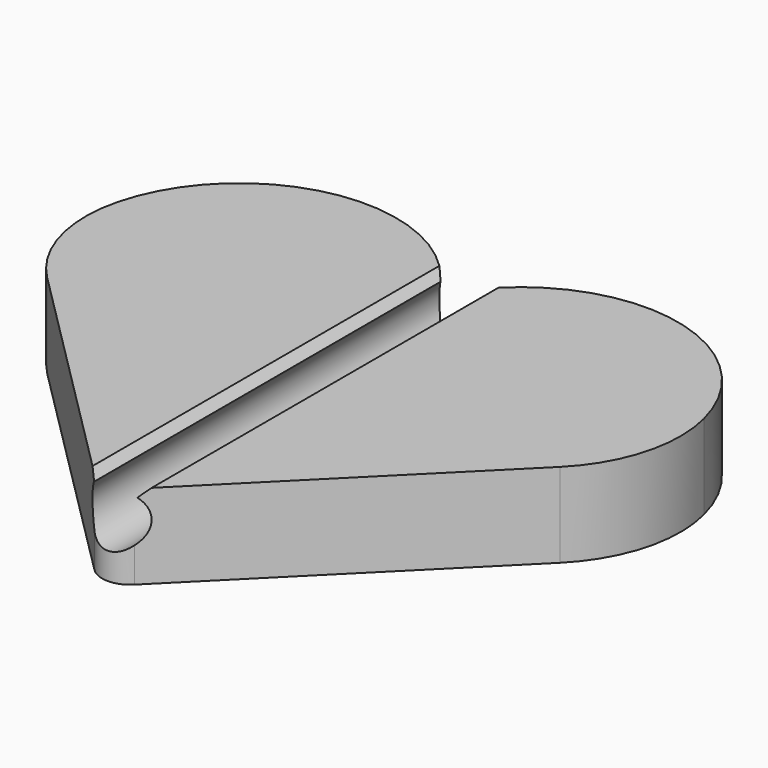
from build123d import *

# Parameters (mm, degrees)
F1_DEPTH      = 3
F2_W          = 4
F2_H          = 6.1803398875
F3_DEPTH      = 1
F5_DEPTH      = 8.0911699437
F5_DEPTH_BACK = 10.001
F6_T1_DEPTH   = 16.9244695544
F7_DEPTH      = 1
F8_R          = 5
F9_R          = 1


# Not quite as in the source:
# - a fillet or chamfer that OpenCascade refuses, or shapes differently, is made with other operations: its cross-section is extruded or revolved along the edge and cut away or added


with BuildPart() as f1:
    # F0 (on Top) → F1 (new body)
    with BuildSketch(Plane.XY):
        with BuildLine():
            ThreePointArc((10, 0), (7.5, 7.5), (0, 5))
            ThreePointArc((0, 5), (-7.5, 7.5), (-10, 0))
            Line((-10, 0), (0, -10))
            Line((0, -10), (10, 0))
        make_face()
    extrude(amount=F1_DEPTH)

    # F2 (on face) → F3 (join)
    with BuildSketch(Plane.XY.offset(3)):
        with BuildLine():
            ThreePointArc((0, 5), (-7.5, 7.5), (-10, 0))
            Line((-10, 0), (0, -10))
            Line((0, -10), (10, 0))
            ThreePointArc((10, 0), (7.5, 7.5), (0, 5))
        make_face()
        Rectangle(F2_W, F2_H, mode=Mode.SUBTRACT)
        Rectangle(F2_W, F2_H)
    extrude(amount=F3_DEPTH)

    # F4 (on Front) → F5 (cut, two sides)
    with BuildSketch(Plane.XZ) as f5_sk:
        with BuildLine():
            Line((0.75, 4), (-0.75, 4))
            Line((-0.75, 4), (-0.75, 3.7348469228))
            ThreePointArc((-0.75, 3.7348469228), (0, 1.95), (0.75, 3.7348469228))
            Line((0.75, 3.7348469228), (0.75, 4))
        make_face()
    extrude(amount=-F5_DEPTH, mode=Mode.SUBTRACT)
    extrude(f5_sk.sketch, amount=F5_DEPTH_BACK, mode=Mode.SUBTRACT)

    # F6: chamfer of 0.3 on 2 edges, made by hand

    # F6_s2 → F6_t1 (cut)
    with BuildSketch(Plane.XZ.offset(-6.902964658)):
        Polygon((1.05, 4), (0.75, 3.7), (0.75, 4), align=None)
        Polygon((-0.75, 3.7), (-1.05, 4), (-0.75, 4), align=None)
    extrude(amount=F6_T1_DEPTH, mode=Mode.SUBTRACT)

    # F7 (cut): a face of the model
    f7_faces = [f1.faces().sort_by_distance(p)[0] for p in [
        (0, 0.8210756438, 0),
    ]]
    extrude(f7_faces, amount=-F7_DEPTH, mode=Mode.SUBTRACT)

    # F8
    f8_edges = [f1.edges().sort_by_distance(p)[0] for p in [
        (10, 0, 2.5),
        (-10, 0, 2.5),
    ]]
    fillet(f8_edges, radius=F8_R)

    # F9
    f9_edges = [f1.edges().sort_by_distance(p)[0] for p in [
        (0, -10, 1.475),
    ]]
    fillet(f9_edges, radius=F9_R)


solid = f1.part
